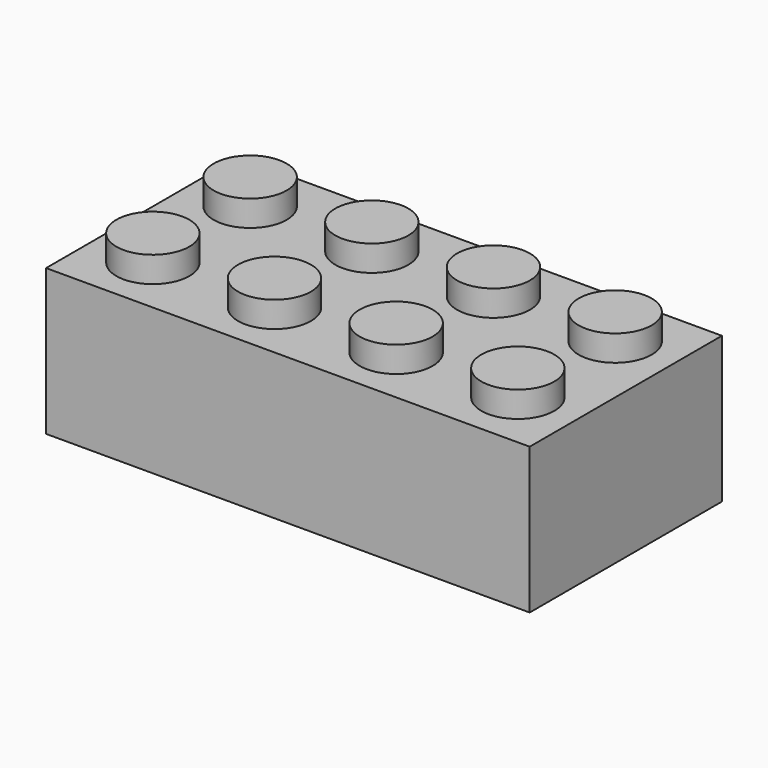
from build123d import *

# Parameters (mm, degrees)
F0_W     = 31.8
F0_H     = 15.8
F0_W_2   = 29.4
F0_H_2   = 13.4
F0_R     = 3.25
F0_R_2   = 2.4
F1_DEPTH = 9.6
F2_DEPTH = 7.9
F3_R     = 2.4
F4_DEPTH = 1.7
F5_W     = 0.6
F5_H     = 0.3
F5_W_2   = 0.3
F5_H_2   = 0.6
F6_DEPTH = 7.9


# Not quite as in the source:
# - a feature names something its author has since deleted; it is built from what else it names


with BuildPart() as f1:
    # F0 (on Top) → F1 (new body)
    with BuildSketch(Plane.XY):
        Rectangle(F0_W, F0_H)
        Rectangle(F0_W_2, F0_H_2, mode=Mode.SUBTRACT)
        Rectangle(F0_W_2, F0_H_2)
        with Locations((-8, 0)):
            Circle(F0_R, mode=Mode.SUBTRACT)
        Circle(F0_R, mode=Mode.SUBTRACT)
        with Locations((8, 0)):
            Circle(F0_R, mode=Mode.SUBTRACT)
        with Locations((-8, 0)):
            Circle(F0_R)
        with Locations((-8, 0)):
            Circle(F0_R_2, mode=Mode.SUBTRACT)
        Circle(F0_R)
        Circle(F0_R_2, mode=Mode.SUBTRACT)
        with Locations((8, 0)):
            Circle(F0_R)
        with Locations((8, 0)):
            Circle(F0_R_2, mode=Mode.SUBTRACT)
        with Locations((-8, 0)):
            Circle(F0_R_2)
        Circle(F0_R_2)
        with Locations((8, 0)):
            Circle(F0_R_2)
    extrude(amount=F1_DEPTH)

    # F0 (on Top) → F2 (cut)
    with BuildSketch(Plane.XY):
        Rectangle(F0_W_2, F0_H_2)
        with Locations((-8, 0)):
            Circle(F0_R, mode=Mode.SUBTRACT)
        Circle(F0_R, mode=Mode.SUBTRACT)
        with Locations((8, 0)):
            Circle(F0_R, mode=Mode.SUBTRACT)
        with Locations((-8, 0)):
            Circle(F0_R_2)
        with Locations((8, 0)):
            Circle(F0_R_2)
        Circle(F0_R_2)
    extrude(amount=F2_DEPTH, mode=Mode.SUBTRACT)

    # F3 (on face) → F4 (join)
    with BuildSketch(Plane.XY.offset(9.6)):
        with Locations((-12, 4)):
            Circle(F3_R)
        with Locations((-12, -4)):
            Circle(F3_R)
        with Locations((-4, 4)):
            Circle(F3_R)
        with Locations((-4, -4)):
            Circle(F3_R)
        with Locations((4, 4)):
            Circle(F3_R)
        with Locations((4, -4)):
            Circle(F3_R)
        with Locations((12, 4)):
            Circle(F3_R)
        with Locations((12, -4)):
            Circle(F3_R)
    extrude(amount=F4_DEPTH)

    # F5 (on Top) → F6 (join, through all)
    with BuildSketch(Plane.XY):
        with Locations((-12, -6.55)):
            Rectangle(F5_W, F5_H)
        with Locations((-4, -6.55)):
            Rectangle(F5_W, F5_H)
        with Locations((-14.55, -4)):
            Rectangle(F5_W_2, F5_H_2)
        with Locations((4, -6.55)):
            Rectangle(F5_W, F5_H)
        with Locations((12, -6.55)):
            Rectangle(F5_W, F5_H)
        with Locations((14.55, -4)):
            Rectangle(F5_W_2, F5_H_2)
        with Locations((-4, 6.55)):
            Rectangle(F5_W, F5_H)
        with Locations((14.55, 4)):
            Rectangle(F5_W_2, F5_H_2)
        with Locations((12, 6.55)):
            Rectangle(F5_W, F5_H)
        with Locations((-12, 6.55)):
            Rectangle(F5_W, F5_H)
        with Locations((-14.55, 4)):
            Rectangle(F5_W_2, F5_H_2)
        with Locations((4, 6.55)):
            Rectangle(F5_W, F5_H)
    extrude(amount=F6_DEPTH)


solid = f1.part
